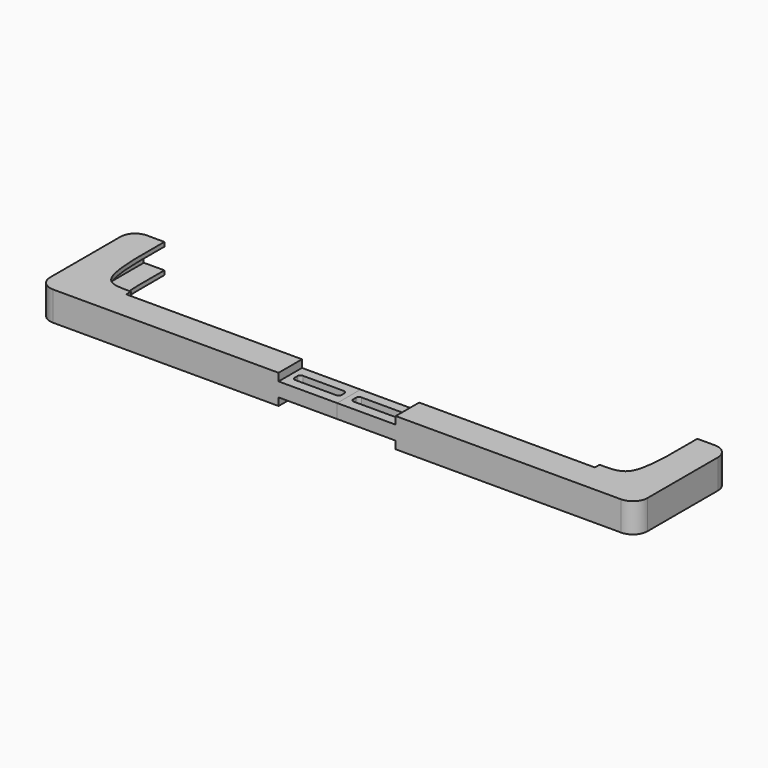
from build123d import *

# Parameters (mm, degrees)
F0_W         = 22
F0_H         = 40
F1_DEPTH     = 5
F2_W         = 18
F2_H         = 7.1
F3_DEPTH     = 28
F4_W         = 10
F4_H         = 10
F5_DEPTH     = 60
F6_W         = 10
F6_H         = 4.8
F7_DEPTH     = 20
F9_DEPTH     = 4.8
F11_DEPTH    = 10
F12_R        = 5
F13_T1_DEPTH = 35


# Not quite as in the source:
# - a fillet or chamfer that OpenCascade refuses, or shapes differently, is made with other operations: its cross-section is extruded or revolved along the edge and cut away or added


with BuildPart() as f1:
    # F0 (on Top) → F1 (new body, symmetric)
    with BuildSketch(Plane.XY):
        Rectangle(F0_W, F0_H)
    extrude(amount=F1_DEPTH, both=True)

    # F2 (on face) → F3 (cut)
    with BuildSketch(Plane(origin=(0, 20, 0), x_dir=(-1, 0, 0), z_dir=(0, 1, 0))):
        with Locations((2, 0)):
            Rectangle(F2_W, F2_H)
    extrude(amount=-F3_DEPTH, mode=Mode.SUBTRACT)

    # F4 (on face) → F5 (join)
    with BuildSketch(Plane(origin=(-11, 0, 0), x_dir=(0, -1, 0), z_dir=(-1, 0, 0))):
        with Locations((15, 0)):
            Rectangle(F4_W, F4_H)
    extrude(amount=F5_DEPTH)

    # F6 (on face) → F7 (join)
    with BuildSketch(Plane(origin=(-71, 0, 0), x_dir=(0, -1, 0), z_dir=(-1, 0, 0))):
        with Locations((15, 0)):
            Rectangle(F6_W, F6_H)
    extrude(amount=F7_DEPTH)

    # F8 (on face) → F9 (cut, through all)
    with BuildSketch(Plane.XY.offset(2.4)):
        with BuildLine():
            Line((-74, -13.4), (-88, -13.4))
            ThreePointArc((-88, -13.4), (-88.7071067812, -13.6928932188), (-89, -14.4))
            Line((-89, -14.4), (-89, -15.6))
            ThreePointArc((-89, -15.6), (-88.7071067812, -16.3071067812), (-88, -16.6))
            Line((-88, -16.6), (-74, -16.6))
            ThreePointArc((-74, -16.6), (-73.2928932188, -16.3071067812), (-73, -15.6))
            Line((-73, -15.6), (-73, -14.4))
            ThreePointArc((-73, -14.4), (-73.2928932188, -13.6928932188), (-74, -13.4))
        make_face()
    extrude(amount=-F9_DEPTH, mode=Mode.SUBTRACT)

    # F10 (on face) → F11 (cut, through all)
    with BuildSketch(Plane.XY.offset(5)):
        with BuildLine():
            add(Edge.make_bspline(
                [(0, 20), (0, 11.0162314684), (0.75924226, -7.767469097), (-6.2310384733, -8), (-11, -8)],
                knots=[0, 0, 0, 0, 0.6211235912, 1, 1, 1, 1], degree=3))
            Line((0, 20), (-11, 20))
            Line((-11, 20), (-11, -8))
        make_face()
    extrude(amount=-F11_DEPTH, mode=Mode.SUBTRACT)

    # F12
    f12_edges = [f1.edges().sort_by_distance(p)[0] for p in [
        (11, -20, 0),
    ]]
    fillet(f12_edges, radius=F12_R)

    # F13: fillet of radius 5 on 1 edges, made by hand

    # F13_s2 → F13_t1 (cut)
    with BuildSketch(Plane.XY.offset(-17.5)):
        with BuildLine():
            ThreePointArc((11, 15), (9.5355339059, 18.5355339059), (6, 20))
            Line((6, 20), (11, 20))
            Line((11, 20), (11, 15))
        make_face()
    extrude(amount=F13_T1_DEPTH, mode=Mode.SUBTRACT)


with BuildPart() as f14_1:
    # F14: instance of F1
    add(f1.part.mirror(Plane(origin=(-91, -15, 0), x_dir=(0, -1, 0), z_dir=(-1, 0, 0))))


solid = Compound([f1.part, f14_1.part])
